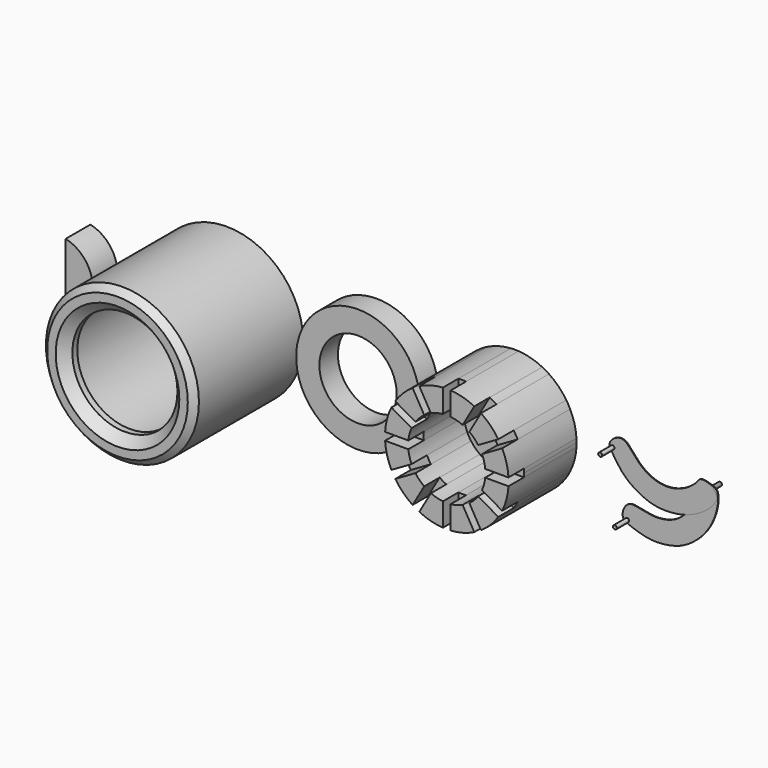
from build123d import *

# Parameters (mm, degrees)
F0_R           = 25.4
F0_R_2         = 0.79375
F0_R_3         = 15.875
F1_DEPTH       = 9.525
F2_START       = 6.35
F2_DEPTH       = 3.175
F3_DEPTH       = 34.925
F4_DEPTH       = 26.9875
F5_DEPTH       = 6.35
F0_R_4         = 31.4325
F0_R_5         = 26.19375
F6_DEPTH       = 0.2667
F7_DEPTH       = 6.35
F7_DEPTH_BACK  = 0.2667
F8_DEPTH       = 6.6167
F9_ANGLE       = -37.4660568631
F10_DEPTH      = 49.7586
F11_DEPTH      = 6.35
F11_DEPTH_BACK = 49.7586
F12_START      = 49.7586
F0_R_6         = 21.59
F12_DEPTH      = 6.35
F13_SIZE       = 3.81
F14_SIZE       = 2.54
F15_DEPTH      = 12.7


# Not quite as in the source:
# - a feature names something its author has since deleted; it is built from what else it names


with BuildPart() as f1:
    # F0 (on Front) → F1 (new body)
    with BuildSketch(Plane.XZ):
        Circle(F0_R)
        with Locations((0, -20.6375)):
            Circle(F0_R_2, mode=Mode.SUBTRACT)
        with Locations((-10.31875, -17.8725992706)):
            Circle(F0_R_2, mode=Mode.SUBTRACT)
        with Locations((-17.8725992706, -10.31875)):
            Circle(F0_R_2, mode=Mode.SUBTRACT)
        with Locations((-20.6375, 0)):
            Circle(F0_R_2, mode=Mode.SUBTRACT)
        Circle(F0_R_3, mode=Mode.SUBTRACT)
        with Locations((10.31875, -17.8725992706)):
            Circle(F0_R_2, mode=Mode.SUBTRACT)
        with Locations((17.8725992706, -10.31875)):
            Circle(F0_R_2, mode=Mode.SUBTRACT)
        with Locations((20.6375, 0)):
            Circle(F0_R_2, mode=Mode.SUBTRACT)
        with Locations((-17.8725992706, 10.31875)):
            Circle(F0_R_2, mode=Mode.SUBTRACT)
        with Locations((-10.31875, 17.8725992706)):
            Circle(F0_R_2, mode=Mode.SUBTRACT)
        with Locations((0, 20.6375)):
            Circle(F0_R_2, mode=Mode.SUBTRACT)
        with Locations((17.8725992706, 10.31875)):
            Circle(F0_R_2, mode=Mode.SUBTRACT)
        with Locations((10.31875, 17.8725992706)):
            Circle(F0_R_2, mode=Mode.SUBTRACT)
    extrude(amount=F1_DEPTH)

    # F0 (on Front) → F2 (join)
    with BuildSketch(Plane.XZ.offset(F2_START)):
        with Locations((0, -20.6375)):
            Circle(F0_R_2)
        with Locations((-10.31875, -17.8725992706)):
            Circle(F0_R_2)
        with Locations((-17.8725992706, -10.31875)):
            Circle(F0_R_2)
        with Locations((-20.6375, 0)):
            Circle(F0_R_2)
        with Locations((-17.8725992706, 10.31875)):
            Circle(F0_R_2)
        with Locations((17.8725992706, 10.31875)):
            Circle(F0_R_2)
        with Locations((20.6375, 0)):
            Circle(F0_R_2)
        with Locations((17.8725992706, -10.31875)):
            Circle(F0_R_2)
        with Locations((10.31875, -17.8725992706)):
            Circle(F0_R_2)
        with Locations((-10.31875, 17.8725992706)):
            Circle(F0_R_2)
        with Locations((0, 20.6375)):
            Circle(F0_R_2)
        with Locations((10.31875, 17.8725992706)):
            Circle(F0_R_2)
    extrude(amount=F2_DEPTH)


with BuildPart() as f3:
    # F0 (on Front) → F3 (new body)
    with BuildSketch(Plane.XZ):
        with BuildLine():
            Line((55.2206624806, 15.7954255641), (55.2206624806, 25.3503420835))
            ThreePointArc((55.2206624806, 25.3503420835), (50.234158735, 24.5345159877), (45.5078067674, 22.7477902389))
            Line((45.5078067674, 22.7477902389), (50.2852650271, 14.4729898021))
            ThreePointArc((50.2852650271, 14.4729898021), (52.6994101396, 15.3340724923), (55.2206624806, 15.7954255641))
        make_face()
    extrude(amount=F3_DEPTH)



with BuildPart() as f3b:
    # F0 (on Front) → F3, piece 2 (new body)
    with BuildSketch(Plane.XZ):
        with BuildLine():
            Line((63.3310599341, 14.4729898021), (68.1085181938, 22.7477902389))
            ThreePointArc((68.1085181938, 22.7477902389), (63.3821662262, 24.5345159877), (58.3956624806, 25.3503420835))
            Line((58.3956624806, 25.3503420835), (58.3956624806, 15.7954255641))
            ThreePointArc((58.3956624806, 15.7954255641), (60.9169148216, 15.3340724923), (63.3310599341, 14.4729898021))
        make_face()
    extrude(amount=F3_DEPTH)


with BuildPart() as f3c:
    # F0 (on Front) → F3, piece 3 (new body)
    with BuildSketch(Plane.XZ):
        with BuildLine():
            Line((69.6936522827, 9.2725281105), (77.9684527195, 14.0499863703))
            ThreePointArc((77.9684527195, 14.0499863703), (74.7686747227, 17.9605122421), (70.8581488508, 21.1602902389))
            Line((70.8581488508, 21.1602902389), (66.0806905911, 12.8854898021))
            ThreePointArc((66.0806905911, 12.8854898021), (68.0334826319, 11.2253201513), (69.6936522827, 9.2725281105))
        make_face()
    extrude(amount=F3_DEPTH)


with BuildPart() as f3d:
    # F0 (on Front) → F3, piece 4 (new body)
    with BuildSketch(Plane.XZ):
        with BuildLine():
            Line((47.5356343701, 12.8854898021), (42.7581761103, 21.1602902389))
            ThreePointArc((42.7581761103, 21.1602902389), (38.8476502385, 17.9605122421), (35.6478722417, 14.0499863703))
            Line((35.6478722417, 14.0499863703), (43.9226726785, 9.2725281105))
            ThreePointArc((43.9226726785, 9.2725281105), (45.5828423293, 11.2253201513), (47.5356343701, 12.8854898021))
        make_face()
    extrude(amount=F3_DEPTH)


with BuildPart() as f3e:
    # F0 (on Front) → F3, piece 5 (new body)
    with BuildSketch(Plane.XZ):
        with BuildLine():
            Line((42.3351726785, 6.5228974535), (34.0603722417, 11.3003557132))
            ThreePointArc((34.0603722417, 11.3003557132), (32.2736464929, 6.5740037456), (31.4578203971, 1.5875))
            Line((31.4578203971, 1.5875), (41.0127369165, 1.5875))
            ThreePointArc((41.0127369165, 1.5875), (41.4740899883, 4.108752341), (42.3351726785, 6.5228974535))
        make_face()
    extrude(amount=F3_DEPTH)


with BuildPart() as f3f:
    # F0 (on Front) → F3, piece 6 (new body)
    with BuildSketch(Plane.XZ):
        with BuildLine():
            ThreePointArc((31.4578203971, -1.5875), (32.2736464929, -6.5740037456), (34.0603722417, -11.3003557132))
            Line((34.0603722417, -11.3003557132), (42.3351726785, -6.5228974535))
            ThreePointArc((42.3351726785, -6.5228974535), (41.4740899883, -4.108752341), (41.0127369165, -1.5875))
            Line((41.0127369165, -1.5875), (31.4578203971, -1.5875))
        make_face()
    extrude(amount=F3_DEPTH)


with BuildPart() as f3g:
    # F0 (on Front) → F3, piece 7 (new body)
    with BuildSketch(Plane.XZ):
        with BuildLine():
            ThreePointArc((35.6478722417, -14.0499863703), (38.8476502385, -17.9605122421), (42.7581761103, -21.1602902389))
            Line((42.7581761103, -21.1602902389), (47.5356343701, -12.8854898021))
            ThreePointArc((47.5356343701, -12.8854898021), (45.5828423293, -11.2253201513), (43.9226726785, -9.2725281105))
            Line((43.9226726785, -9.2725281105), (35.6478722417, -14.0499863703))
        make_face()
    extrude(amount=F3_DEPTH)


with BuildPart() as f3h:
    # F0 (on Front) → F3, piece 8 (new body)
    with BuildSketch(Plane.XZ):
        with BuildLine():
            ThreePointArc((45.5078067674, -22.7477902389), (50.234158735, -24.5345159877), (55.2206624806, -25.3503420835))
            Line((55.2206624806, -25.3503420835), (55.2206624806, -15.7954255641))
            ThreePointArc((55.2206624806, -15.7954255641), (52.6994101396, -15.3340724923), (50.2852650271, -14.4729898021))
            Line((50.2852650271, -14.4729898021), (45.5078067674, -22.7477902389))
        make_face()
    extrude(amount=F3_DEPTH)


with BuildPart() as f3i:
    # F0 (on Front) → F3, piece 9 (new body)
    with BuildSketch(Plane.XZ):
        with BuildLine():
            ThreePointArc((58.3956624806, -25.3503420835), (63.3821662262, -24.5345159877), (68.1085181938, -22.7477902389))
            Line((68.1085181938, -22.7477902389), (63.3310599341, -14.4729898021))
            ThreePointArc((63.3310599341, -14.4729898021), (60.9169148216, -15.3340724923), (58.3956624806, -15.7954255641))
            Line((58.3956624806, -15.7954255641), (58.3956624806, -25.3503420835))
        make_face()
    extrude(amount=F3_DEPTH)


with BuildPart() as f3j:
    # F0 (on Front) → F3, piece 10 (new body)
    with BuildSketch(Plane.XZ):
        with BuildLine():
            ThreePointArc((70.8581488508, -21.1602902389), (74.7686747227, -17.9605122421), (77.9684527195, -14.0499863703))
            Line((77.9684527195, -14.0499863703), (69.6936522827, -9.2725281105))
            ThreePointArc((69.6936522827, -9.2725281105), (68.0334826319, -11.2253201513), (66.0806905911, -12.8854898021))
            Line((66.0806905911, -12.8854898021), (70.8581488508, -21.1602902389))
        make_face()
    extrude(amount=F3_DEPTH)


with BuildPart() as f3k:
    # F0 (on Front) → F3, piece 11 (new body)
    with BuildSketch(Plane.XZ):
        with BuildLine():
            ThreePointArc((79.5559527195, -11.3003557132), (81.3426784683, -6.5740037456), (82.1585045641, -1.5875))
            Line((82.1585045641, -1.5875), (72.6035880447, -1.5875))
            ThreePointArc((72.6035880447, -1.5875), (72.1422349729, -4.108752341), (71.2811522827, -6.5228974535))
            Line((71.2811522827, -6.5228974535), (79.5559527195, -11.3003557132))
        make_face()
    extrude(amount=F3_DEPTH)


with BuildPart() as f3l:
    # F0 (on Front) → F3, piece 12 (new body)
    with BuildSketch(Plane.XZ):
        with BuildLine():
            Line((72.6035880447, 1.5875), (82.1585045641, 1.5875))
            ThreePointArc((82.1585045641, 1.5875), (81.3426784683, 6.5740037456), (79.5559527195, 11.3003557132))
            Line((79.5559527195, 11.3003557132), (71.2811522827, 6.5228974535))
            ThreePointArc((71.2811522827, 6.5228974535), (72.1422349729, 4.108752341), (72.6035880447, 1.5875))
        make_face()
    extrude(amount=F3_DEPTH)


with BuildPart() as f3_1:
    add(f3.part)

    add(f3b.part)  # F4 merges F3b

    add(f3c.part)  # F4 merges F3c

    add(f3d.part)  # F4 merges F3d

    add(f3e.part)  # F4 merges F3e

    add(f3f.part)  # F4 merges F3f

    add(f3g.part)  # F4 merges F3g

    add(f3h.part)  # F4 merges F3h

    add(f3i.part)  # F4 merges F3i

    add(f3j.part)  # F4 merges F3j

    add(f3k.part)  # F4 merges F3k

    add(f3l.part)  # F4 merges F3l
    # F0 (on Front) → F4 (join)
    with BuildSketch(Plane.XZ):
        with BuildLine():
            Line((58.3956624806, 15.7954255641), (58.3956624806, 25.3503420835))
            ThreePointArc((58.3956624806, 25.3503420835), (56.8081624806, 25.4), (55.2206624806, 25.3503420835))
            Line((55.2206624806, 25.3503420835), (55.2206624806, 15.7954255641))
            ThreePointArc((55.2206624806, 15.7954255641), (56.8081624806, 15.875), (58.3956624806, 15.7954255641))
        make_face()
        with BuildLine():
            Line((66.0806905911, 12.8854898021), (70.8581488508, 21.1602902389))
            ThreePointArc((70.8581488508, 21.1602902389), (69.5081624806, 21.9970452561), (68.1085181938, 22.7477902389))
            Line((68.1085181938, 22.7477902389), (63.3310599341, 14.4729898021))
            ThreePointArc((63.3310599341, 14.4729898021), (64.7456624806, 13.7481532851), (66.0806905911, 12.8854898021))
        make_face()
        with BuildLine():
            Line((71.2811522827, 6.5228974535), (79.5559527195, 11.3003557132))
            ThreePointArc((79.5559527195, 11.3003557132), (78.8052077367, 12.7), (77.9684527195, 14.0499863703))
            Line((77.9684527195, 14.0499863703), (69.6936522827, 9.2725281105))
            ThreePointArc((69.6936522827, 9.2725281105), (70.5563157657, 7.9375), (71.2811522827, 6.5228974535))
        make_face()
        with BuildLine():
            ThreePointArc((82.1585045641, -1.5875), (82.1957449661, -0.7941382371), (82.2081624806, 0))
            ThreePointArc((82.2081624806, 0), (82.1957449661, 0.7941382371), (82.1585045641, 1.5875))
            Line((82.1585045641, 1.5875), (72.6035880447, 1.5875))
            ThreePointArc((72.6035880447, 1.5875), (72.6632563912, 0.7947465541), (72.6831624806, 0))
            ThreePointArc((72.6831624806, 0), (72.6632563912, -0.7947465541), (72.6035880447, -1.5875))
            Line((72.6035880447, -1.5875), (82.1585045641, -1.5875))
        make_face()
        with BuildLine():
            Line((43.9226726785, 9.2725281105), (35.6478722417, 14.0499863703))
            ThreePointArc((35.6478722417, 14.0499863703), (34.8111172245, 12.7), (34.0603722417, 11.3003557132))
            Line((34.0603722417, 11.3003557132), (42.3351726785, 6.5228974535))
            ThreePointArc((42.3351726785, 6.5228974535), (43.0600091955, 7.9375), (43.9226726785, 9.2725281105))
        make_face()
        with BuildLine():
            Line((50.2852650271, 14.4729898021), (45.5078067674, 22.7477902389))
            ThreePointArc((45.5078067674, 22.7477902389), (44.1081624806, 21.9970452561), (42.7581761103, 21.1602902389))
            Line((42.7581761103, 21.1602902389), (47.5356343701, 12.8854898021))
            ThreePointArc((47.5356343701, 12.8854898021), (48.8706624806, 13.7481532851), (50.2852650271, 14.4729898021))
        make_face()
        with BuildLine():
            Line((41.0127369165, 1.5875), (31.4578203971, 1.5875))
            ThreePointArc((31.4578203971, 1.5875), (31.4081624806, 0), (31.4578203971, -1.5875))
            Line((31.4578203971, -1.5875), (41.0127369165, -1.5875))
            ThreePointArc((41.0127369165, -1.5875), (40.9331624806, 0), (41.0127369165, 1.5875))
        make_face()
        with BuildLine():
            ThreePointArc((77.9684527195, -14.0499863703), (78.8052077367, -12.7), (79.5559527195, -11.3003557132))
            Line((79.5559527195, -11.3003557132), (71.2811522827, -6.5228974535))
            ThreePointArc((71.2811522827, -6.5228974535), (70.5563157657, -7.9375), (69.6936522827, -9.2725281105))
            Line((69.6936522827, -9.2725281105), (77.9684527195, -14.0499863703))
        make_face()
        with BuildLine():
            ThreePointArc((34.0603722417, -11.3003557132), (34.8111172245, -12.7), (35.6478722417, -14.0499863703))
            Line((35.6478722417, -14.0499863703), (43.9226726785, -9.2725281105))
            ThreePointArc((43.9226726785, -9.2725281105), (43.0600091955, -7.9375), (42.3351726785, -6.5228974535))
            Line((42.3351726785, -6.5228974535), (34.0603722417, -11.3003557132))
        make_face()
        with BuildLine():
            ThreePointArc((42.7581761103, -21.1602902389), (44.1081624806, -21.9970452561), (45.5078067674, -22.7477902389))
            Line((45.5078067674, -22.7477902389), (50.2852650271, -14.4729898021))
            ThreePointArc((50.2852650271, -14.4729898021), (48.8706624806, -13.7481532851), (47.5356343701, -12.8854898021))
            Line((47.5356343701, -12.8854898021), (42.7581761103, -21.1602902389))
        make_face()
        with BuildLine():
            ThreePointArc((55.2206624806, -25.3503420835), (56.8081624806, -25.4), (58.3956624806, -25.3503420835))
            Line((58.3956624806, -25.3503420835), (58.3956624806, -15.7954255641))
            ThreePointArc((58.3956624806, -15.7954255641), (56.8081624806, -15.875), (55.2206624806, -15.7954255641))
            Line((55.2206624806, -15.7954255641), (55.2206624806, -25.3503420835))
        make_face()
        with BuildLine():
            ThreePointArc((68.1085181938, -22.7477902389), (69.5081624806, -21.9970452561), (70.8581488508, -21.1602902389))
            Line((70.8581488508, -21.1602902389), (66.0806905911, -12.8854898021))
            ThreePointArc((66.0806905911, -12.8854898021), (64.7456624806, -13.7481532851), (63.3310599341, -14.4729898021))
            Line((63.3310599341, -14.4729898021), (68.1085181938, -22.7477902389))
        make_face()
    extrude(amount=F4_DEPTH)

    # F0 (on Front) → F5 (join)
    with BuildSketch(Plane.XZ):
        with BuildLine():
            ThreePointArc((72.6831624806, 0), (72.6632563912, 0.7947465541), (72.6035880447, 1.5875))
            ThreePointArc((72.6035880447, 1.5875), (72.1422349729, 4.108752341), (71.2811522827, 6.5228974535))
            ThreePointArc((71.2811522827, 6.5228974535), (70.5563157657, 7.9375), (69.6936522827, 9.2725281105))
            ThreePointArc((69.6936522827, 9.2725281105), (68.0334826319, 11.2253201513), (66.0806905911, 12.8854898021))
            ThreePointArc((66.0806905911, 12.8854898021), (64.7456624806, 13.7481532851), (63.3310599341, 14.4729898021))
            ThreePointArc((63.3310599341, 14.4729898021), (60.9169148216, 15.3340724923), (58.3956624806, 15.7954255641))
            ThreePointArc((58.3956624806, 15.7954255641), (56.8081624806, 15.875), (55.2206624806, 15.7954255641))
            ThreePointArc((55.2206624806, 15.7954255641), (52.6994101396, 15.3340724923), (50.2852650271, 14.4729898021))
            ThreePointArc((50.2852650271, 14.4729898021), (48.8706624806, 13.7481532851), (47.5356343701, 12.8854898021))
            ThreePointArc((47.5356343701, 12.8854898021), (45.5828423293, 11.2253201513), (43.9226726785, 9.2725281105))
            ThreePointArc((43.9226726785, 9.2725281105), (43.0600091955, 7.9375), (42.3351726785, 6.5228974535))
            ThreePointArc((42.3351726785, 6.5228974535), (41.4740899883, 4.108752341), (41.0127369165, 1.5875))
            ThreePointArc((41.0127369165, 1.5875), (40.9331624806, 0), (41.0127369165, -1.5875))
            ThreePointArc((41.0127369165, -1.5875), (41.4740899883, -4.108752341), (42.3351726785, -6.5228974535))
            ThreePointArc((42.3351726785, -6.5228974535), (43.0600091955, -7.9375), (43.9226726785, -9.2725281105))
            ThreePointArc((43.9226726785, -9.2725281105), (45.5828423293, -11.2253201513), (47.5356343701, -12.8854898021))
            ThreePointArc((47.5356343701, -12.8854898021), (48.8706624806, -13.7481532851), (50.2852650271, -14.4729898021))
            ThreePointArc((50.2852650271, -14.4729898021), (52.6994101396, -15.3340724923), (55.2206624806, -15.7954255641))
            ThreePointArc((55.2206624806, -15.7954255641), (56.8081624806, -15.875), (58.3956624806, -15.7954255641))
            ThreePointArc((58.3956624806, -15.7954255641), (60.9169148216, -15.3340724923), (63.3310599341, -14.4729898021))
            ThreePointArc((63.3310599341, -14.4729898021), (64.7456624806, -13.7481532851), (66.0806905911, -12.8854898021))
            ThreePointArc((66.0806905911, -12.8854898021), (68.0334826319, -11.2253201513), (69.6936522827, -9.2725281105))
            ThreePointArc((69.6936522827, -9.2725281105), (70.5563157657, -7.9375), (71.2811522827, -6.5228974535))
            ThreePointArc((71.2811522827, -6.5228974535), (72.1422349729, -4.108752341), (72.6035880447, -1.5875))
            ThreePointArc((72.6035880447, -1.5875), (72.6632563912, -0.7947465541), (72.6831624806, 0))
        make_face()
    extrude(amount=F5_DEPTH)


with BuildPart() as f5:
    # F0 (on Front) → F5, piece 2 (new body)
    with BuildSketch(Plane.XZ):
        with Locations((-61.5494474769, 0)):
            Circle(F0_R_4)
        with Locations((-61.5494474769, 0)):
            Circle(F0_R_5, mode=Mode.SUBTRACT)
    extrude(amount=F5_DEPTH)



with BuildPart() as f6:
    # F0 (on Front) → F6 (new body)
    with BuildSketch(Plane.XZ):
        with BuildLine():
            ThreePointArc((102.3482280424, -21.7871143528), (102.5262313453, -21.8928069421), (102.7050901532, -21.9970452561))
            add(Edge.make_bspline(
                [(140.2999311686, 0.9983701166), (141.1751806736, -2.5787407067), (138.3772261252, -13.5671555234), (128.4425691897, -22.1258436917), (122.1098849158, -24.4421553787), (114.5736074319, -25.503540019), (108.8216055703, -24.5319736415), (102.7050901532, -21.9970452561)],
                knots=[0, 0, 0, 0, 0.2320799138, 0.4564495916, 0.6153284094, 0.7750758821, 1, 1, 1, 1], degree=3))
            add(Edge.make_bspline(
                [(140.2999311686, 0.9983701166), (140.0760497177, 1.9578481445), (135.8573465785, 4.5323263879), (131.4320635794, 1.3877124827), (131.547421217, 0.5417172215)],
                knots=[0, 0, 0, 0, 0.4997315761, 1, 1, 1, 1], degree=3))
            add(Edge.make_bspline(
                [(104.1102409363, -15.0225190446), (105.0013236076, -14.4994918264), (108.296186489, -15.1356276759), (115.5929560373, -16.9005135886), (126.4431106898, -14.185179302), (131.5156311531, -5.2435880903), (131.547421217, 0.5417172215)],
                knots=[0, 0, 0, 0, 0.1657862571, 0.3995097974, 0.6718590469, 1, 1, 1, 1], degree=3))
            add(Edge.make_bspline(
                [(104.1102409363, -15.0225190446), (101.9554383537, -15.535567955), (100.1207523979, -20.2013937323), (102.3482280424, -21.7871143528)],
                knots=[0, 0, 0, 0, 6.782557689, 6.782557689, 6.782557689, 6.782557689], degree=3))
        make_face()
        with Locations((103.2342568199, -21.0805017038)):
            Circle(F0_R_2, mode=Mode.SUBTRACT)
        with Locations((136.0425901532, 0)):
            Circle(F0_R_2, mode=Mode.SUBTRACT)
    extrude(amount=F6_DEPTH)

    # F0 (on Front) → F7 (join, two sides)
    with BuildSketch(Plane.XZ) as f7_sk:
        with Locations((136.0425901532, 0)):
            Circle(F0_R_2)
    extrude(amount=-F7_DEPTH)
    extrude(f7_sk.sketch, amount=F7_DEPTH_BACK)

    # F0 (on Front) → F8 (join)
    with BuildSketch(Plane.XZ):
        with Locations((103.2342568199, -21.0805017038)):
            Circle(F0_R_2)
    extrude(amount=F8_DEPTH)


with BuildPart() as f9_1:
    # F9: copy of F6
    add(f6.part.rotate(Axis((136.0425901532, 0, 0), (0, -1, 0)), F9_ANGLE))


with BuildPart() as f10:
    # F0 (on Front) → F10 (new body)
    with BuildSketch(Plane.XZ):
        with Locations((-61.5494474769, 0)):
            Circle(F0_R_4)
        with Locations((-61.5494474769, 0)):
            Circle(F0_R_5, mode=Mode.SUBTRACT)
    extrude(amount=F10_DEPTH)


with BuildPart() as f5_1:
    add(f5.part)
    # F11 (add, two sides): a face of the model
    f11_faces = [f10.part.faces().sort_by_distance(p)[0] for p in [
        (-92.0929021209, -49.7586, 0),
    ]]

    add(f10.part)  # F11 merges F10
    extrude(f11_faces, amount=F11_DEPTH)
    extrude(f11_faces, amount=-F11_DEPTH_BACK)

    # F0 (on Front) → F12 (join)
    with BuildSketch(Plane.XZ.offset(F12_START)):
        with Locations((-61.5494474769, 0)):
            Circle(F0_R_5)
        with Locations((-61.5494474769, 0)):
            Circle(F0_R_6, mode=Mode.SUBTRACT)
    extrude(amount=F12_DEPTH)

    # F13
    f13_edges = [f5_1.edges().sort_by_distance(p)[0] for p in [
        (-83.139447, -56.1086, 0),
    ]]
    chamfer(f13_edges, length=F13_SIZE)

    # F14
    f14_edges = [f5_1.edges().sort_by_distance(p)[0] for p in [
        (-92.981947, -56.1086, 0),
    ]]
    chamfer(f14_edges, length=F14_SIZE)


with BuildPart() as f15:
    # F0 (on Front) → F15 (new body)
    with BuildSketch(Plane.XZ):
        with BuildLine():
            ThreePointArc((-117.572692883, -13.930255965), (-109.5786403549, -8.9098216523), (-106.460192883, 0))
            ThreePointArc((-106.460192883, 0), (-109.5786403549, 8.9098216523), (-117.572692883, 13.930255965))
            Line((-117.572692883, 13.930255965), (-117.572692883, -13.930255965))
        make_face()
    extrude(amount=F15_DEPTH)


solid = Compound([f1.part, f3_1.part, f6.part, f9_1.part, f5_1.part, f15.part])
